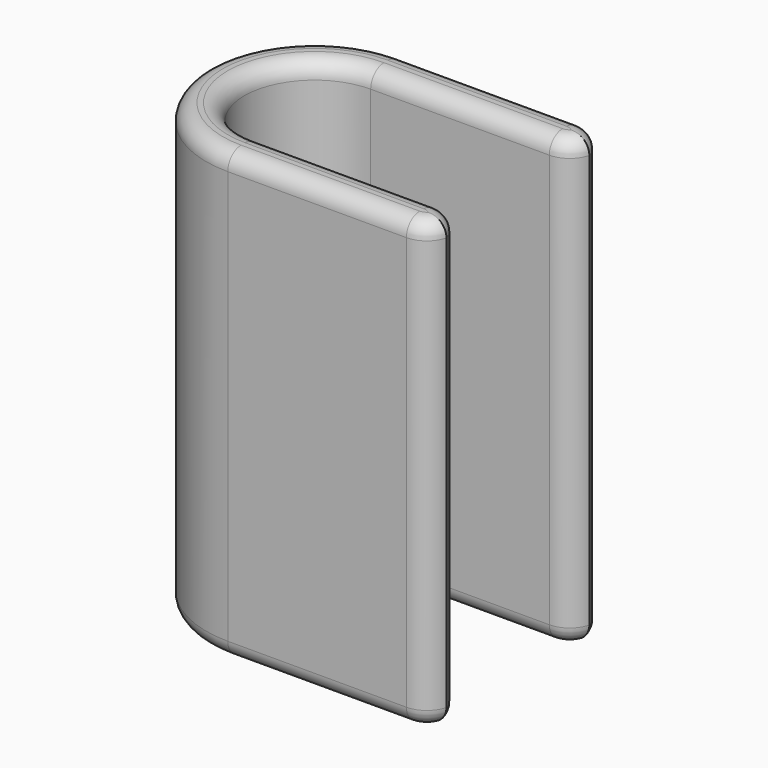
from build123d import *

# Parameters (mm, degrees)
F1_DEPTH     = 17.5
F2_T1_DEPTH  = 22.5
F3_T1_DEPTH  = 7
F3_T4_ANGLE  = 168.6544636073
F3_T6_ANGLE  = 168.6544636073
F3_T8_ANGLE  = 180
F3_T10_ANGLE = 168.6544636073
F3_T12_ANGLE = 168.6544636073
F3_T14_ANGLE = 180
F3_T16_ANGLE = 168.6544636073
F3_T18_ANGLE = 168.6544636073
F3_T20_ANGLE = 180
F3_T22_ANGLE = 168.6544636073
F3_T24_ANGLE = 168.6544636073
F3_T26_ANGLE = 180


# Not quite as in the source:
# - a fillet or chamfer that OpenCascade refuses, or shapes differently, is made with other operations: its cross-section is extruded or revolved along the edge and cut away or added


with BuildPart() as f1:
    # F0 (on Top) → F1 (new body)
    with BuildSketch(Plane.XY):
        with BuildLine():
            ThreePointArc((0, -2.75), (-2.75, 0), (0, 2.75))
            Line((0, 2.75), (8, 2.75))
            Line((8, 2.75), (8, 4.25))
            Line((8, 4.25), (0, 4.25))
            ThreePointArc((0, 4.25), (-4.25, 0), (0, -4.25))
            Line((0, -4.25), (8, -4.25))
            Line((8, -4.25), (8, -2.75))
            Line((8, -2.75), (0, -2.75))
        make_face()
    extrude(amount=F1_DEPTH)

    # F2: fillet of radius 1 on 4 edges, made by hand

    # F2_s2 → F2_t1 (cut)
    with BuildSketch(Plane.XY.offset(-2.5)):
        with BuildLine():
            ThreePointArc((8, -3.75), (7.7071067812, -3.0428932188), (7, -2.75))
            Line((7, -2.75), (8, -2.75))
            Line((8, -2.75), (8, -3.75))
        make_face()
        with BuildLine():
            ThreePointArc((7, -4.25), (7.7071067812, -3.9571067812), (8, -3.25))
            Line((8, -3.25), (8, -4.25))
            Line((8, -4.25), (7, -4.25))
        make_face()
        with BuildLine():
            ThreePointArc((7, 2.75), (7.7071067812, 3.0428932188), (8, 3.75))
            Line((8, 3.75), (8, 2.75))
            Line((8, 2.75), (7, 2.75))
        make_face()
        with BuildLine():
            ThreePointArc((8, 3.25), (7.7071067812, 3.9571067812), (7, 4.25))
            Line((7, 4.25), (8, 4.25))
            Line((8, 4.25), (8, 3.25))
        make_face()
    extrude(amount=F2_T1_DEPTH, mode=Mode.SUBTRACT)

    # F3: fillet of radius 0.65 on 20 edges, made by hand

    # F3_s2 → F3_t1 (cut)
    with BuildSketch(Plane.YZ):
        with BuildLine():
            ThreePointArc((-2.75, 0.65), (-2.9403805922, 0.1903805922), (-3.4, 0))
            Line((-3.4, 0), (-2.75, 0))
            Line((-2.75, 0), (-2.75, 0.65))
        make_face()
        with BuildLine():
            ThreePointArc((-3.6, 0), (-4.0596194078, 0.1903805922), (-4.25, 0.65))
            Line((-4.25, 0.65), (-4.25, 0))
            Line((-4.25, 0), (-3.6, 0))
        make_face()
        with BuildLine():
            ThreePointArc((3.6, 0), (4.0596194078, 0.1903805922), (4.25, 0.65))
            Line((4.25, 0.65), (4.25, 0))
            Line((4.25, 0), (3.6, 0))
        make_face()
        with BuildLine():
            ThreePointArc((2.75, 0.65), (2.9403805922, 0.1903805922), (3.4, 0))
            Line((3.4, 0), (2.75, 0))
            Line((2.75, 0), (2.75, 0.65))
        make_face()
        with BuildLine():
            ThreePointArc((-2.75, 16.85), (-2.9403805922, 17.3096194078), (-3.4, 17.5))
            Line((-3.4, 17.5), (-2.75, 17.5))
            Line((-2.75, 17.5), (-2.75, 16.85))
        make_face()
        with BuildLine():
            ThreePointArc((-3.6, 17.5), (-4.0596194078, 17.3096194078), (-4.25, 16.85))
            Line((-4.25, 16.85), (-4.25, 17.5))
            Line((-4.25, 17.5), (-3.6, 17.5))
        make_face()
        with BuildLine():
            ThreePointArc((3.6, 17.5), (4.0596194078, 17.3096194078), (4.25, 16.85))
            Line((4.25, 16.85), (4.25, 17.5))
            Line((4.25, 17.5), (3.6, 17.5))
        make_face()
        with BuildLine():
            ThreePointArc((2.75, 16.85), (2.9403805922, 17.3096194078), (3.4, 17.5))
            Line((3.4, 17.5), (2.75, 17.5))
            Line((2.75, 17.5), (2.75, 16.85))
        make_face()
    extrude(amount=F3_T1_DEPTH, mode=Mode.SUBTRACT)

    # F3_s3 → F3_t4 (revolve, cut)
    with BuildSketch(Plane.YZ.offset(7)):
        with BuildLine():
            ThreePointArc((-3.4, 0), (-2.9403805922, 0.1903805922), (-2.75, 0.65))
            Line((-2.75, 0.65), (-2.75, 0))
            Line((-2.75, 0), (-3.4, 0))
        make_face()
    revolve(axis=Axis((7, -3.75, 0), (0, 0, -1)), revolution_arc=F3_T4_ANGLE, mode=Mode.SUBTRACT)

    # F3_s5 → F3_t6 (revolve, cut)
    with BuildSketch(Plane(origin=(7.3559574547, -1.4759459573, 0), x_dir=(0, 0, 1), z_dir=(-0.9804586187, 0.1967254356, 0))):
        with BuildLine():
            ThreePointArc((0, -1.4594124616), (0.1903805922, -0.9997930538), (0.65, -0.8094124616))
            Line((0.65, -0.8094124616), (0, -0.8094124616))
            Line((0, -0.8094124616), (0, -1.4594124616))
        make_face()
    revolve(axis=Axis((7, -3.25, 0), (0, 0, -1)), revolution_arc=F3_T6_ANGLE, mode=Mode.SUBTRACT)

    # F3_s7 → F3_t8 (revolve, cut)
    with BuildSketch(Plane.YZ):
        with BuildLine():
            ThreePointArc((3.6, 0), (4.0596194078, 0.1903805922), (4.25, 0.65))
            Line((4.25, 0.65), (4.25, 0))
            Line((4.25, 0), (3.6, 0))
        make_face()
    revolve(axis=Axis((0, 0, 0), (0, 0, 1)), revolution_arc=F3_T8_ANGLE, mode=Mode.SUBTRACT)

    # F3_s9 → F3_t10 (revolve, cut)
    with BuildSketch(Plane.YZ.offset(7)):
        with BuildLine():
            ThreePointArc((3.6, 0), (4.0596194078, 0.1903805922), (4.25, 0.65))
            Line((4.25, 0.65), (4.25, 0))
            Line((4.25, 0), (3.6, 0))
        make_face()
    revolve(axis=Axis((7, 3.25, 0), (0, 0, -1)), revolution_arc=F3_T10_ANGLE, mode=Mode.SUBTRACT)

    # F3_s11 → F3_t12 (revolve, cut)
    with BuildSketch(Plane(origin=(6.0057894127, -1.2050396782, 0), x_dir=(0, 0, 1), z_dir=(-0.9804586187, 0.1967254356, 0))):
        with BuildLine():
            ThreePointArc((0, 5.4037978693), (0.1903805922, 5.8634172771), (0.65, 6.0537978693))
            Line((0.65, 6.0537978693), (0, 6.0537978693))
            Line((0, 6.0537978693), (0, 5.4037978693))
        make_face()
    revolve(axis=Axis((7, 3.75, 0), (0, 0, -1)), revolution_arc=F3_T12_ANGLE, mode=Mode.SUBTRACT)

    # F3_s13 → F3_t14 (revolve, cut)
    with BuildSketch(Plane.YZ):
        with BuildLine():
            ThreePointArc((-2.75, 0.65), (-2.9403805922, 0.1903805922), (-3.4, 0))
            Line((-3.4, 0), (-2.75, 0))
            Line((-2.75, 0), (-2.75, 0.65))
        make_face()
    revolve(axis=Axis((0, 0, 0), (0, 0, -1)), revolution_arc=F3_T14_ANGLE, mode=Mode.SUBTRACT)

    # F3_s15 → F3_t16 (revolve, cut)
    with BuildSketch(Plane.YZ.offset(7)):
        with BuildLine():
            ThreePointArc((-3.4, 17.5), (-2.9403805922, 17.3096194078), (-2.75, 16.85))
            Line((-2.75, 16.85), (-2.75, 17.5))
            Line((-2.75, 17.5), (-3.4, 17.5))
        make_face()
    revolve(axis=Axis((7, -3.75, 17.5), (0, 0, -1)), revolution_arc=F3_T16_ANGLE, mode=Mode.SUBTRACT)

    # F3_s17 → F3_t18 (revolve, cut)
    with BuildSketch(Plane(origin=(7.3559574547, -1.4759459573, 0), x_dir=(0, 0, 1), z_dir=(-0.9804586187, 0.1967254356, 0))):
        with BuildLine():
            ThreePointArc((17.5, -1.4594124616), (17.3096194078, -0.9997930538), (16.85, -0.8094124616))
            Line((16.85, -0.8094124616), (17.5, -0.8094124616))
            Line((17.5, -0.8094124616), (17.5, -1.4594124616))
        make_face()
    revolve(axis=Axis((7, -3.25, 17.5), (0, 0, -1)), revolution_arc=F3_T18_ANGLE, mode=Mode.SUBTRACT)

    # F3_s19 → F3_t20 (revolve, cut)
    with BuildSketch(Plane.YZ):
        with BuildLine():
            ThreePointArc((3.6, 17.5), (4.0596194078, 17.3096194078), (4.25, 16.85))
            Line((4.25, 16.85), (4.25, 17.5))
            Line((4.25, 17.5), (3.6, 17.5))
        make_face()
    revolve(axis=Axis((0, 0, 17.5), (0, 0, 1)), revolution_arc=F3_T20_ANGLE, mode=Mode.SUBTRACT)

    # F3_s21 → F3_t22 (revolve, cut)
    with BuildSketch(Plane.YZ.offset(7)):
        with BuildLine():
            ThreePointArc((3.6, 17.5), (4.0596194078, 17.3096194078), (4.25, 16.85))
            Line((4.25, 16.85), (4.25, 17.5))
            Line((4.25, 17.5), (3.6, 17.5))
        make_face()
    revolve(axis=Axis((7, 3.25, 17.5), (0, 0, -1)), revolution_arc=F3_T22_ANGLE, mode=Mode.SUBTRACT)

    # F3_s23 → F3_t24 (revolve, cut)
    with BuildSketch(Plane(origin=(6.0057894127, -1.2050396782, 0), x_dir=(0, 0, 1), z_dir=(-0.9804586187, 0.1967254356, 0))):
        with BuildLine():
            ThreePointArc((17.5, 5.4037978693), (17.3096194078, 5.8634172771), (16.85, 6.0537978693))
            Line((16.85, 6.0537978693), (17.5, 6.0537978693))
            Line((17.5, 6.0537978693), (17.5, 5.4037978693))
        make_face()
    revolve(axis=Axis((7, 3.75, 17.5), (0, 0, -1)), revolution_arc=F3_T24_ANGLE, mode=Mode.SUBTRACT)

    # F3_s25 → F3_t26 (revolve, cut)
    with BuildSketch(Plane.YZ):
        with BuildLine():
            ThreePointArc((-2.75, 16.85), (-2.9403805922, 17.3096194078), (-3.4, 17.5))
            Line((-3.4, 17.5), (-2.75, 17.5))
            Line((-2.75, 17.5), (-2.75, 16.85))
        make_face()
    revolve(axis=Axis((0, 0, 17.5), (0, 0, -1)), revolution_arc=F3_T26_ANGLE, mode=Mode.SUBTRACT)


solid = f1.part
